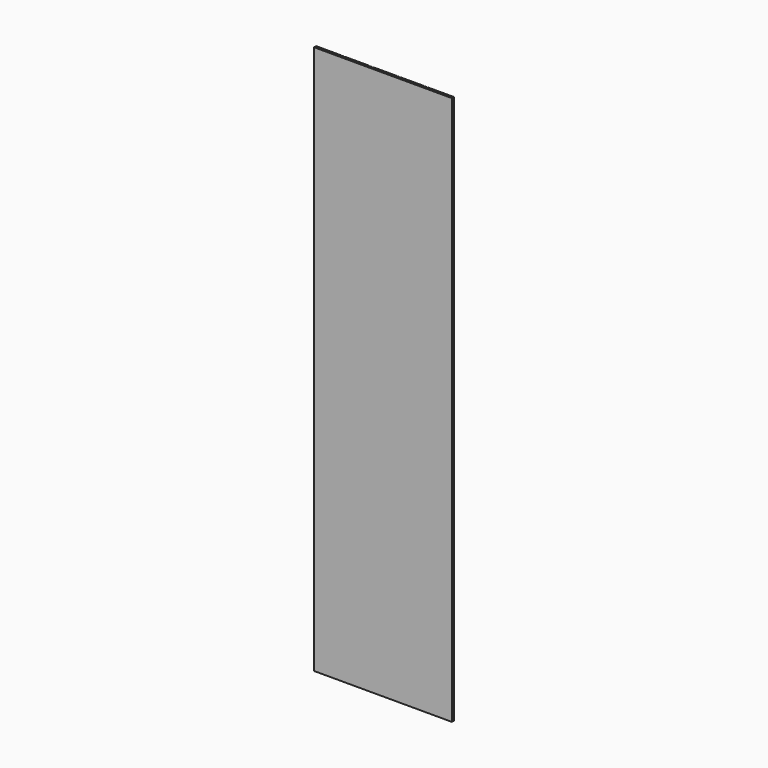
from build123d import *

# Parameters (mm, degrees)
F1_DEPTH = 2390


# Not quite as in the source:
# - a feature names something its author has since deleted; it is built from what else it names


with BuildPart() as f1:
    # F0 (on Top) → F1 (new body)
    with BuildSketch(Plane.XY):
        with BuildLine():
            Line((-309.5, -5.5), (290.5, -5.5))
            ThreePointArc((290.5, -5.5), (285, 0), (290.5, 5.5))
            Line((290.5, 5.5), (180.5, 5.5))
            Line((180.5, 5.5), (176, 0))
            ThreePointArc((176, 0), (170.5, 5.5), (165, 0))
            Line((165, 0), (160.5, 5.5))
            Line((160.5, 5.5), (60.5, 5.5))
            Line((60.5, 5.5), (56, 0))
            ThreePointArc((56, 0), (54.3890872965, 3.8890872965), (50.5, 5.5))
            ThreePointArc((50.5, 5.5), (46.6109127035, 3.8890872965), (45, 0))
            Line((45, 0), (40.5, 5.5))
            Line((40.5, 5.5), (-59.5, 5.5))
            Line((-59.5, 5.5), (-64, 0))
            ThreePointArc((-64, 0), (-65.6109127035, 3.8890872965), (-69.5, 5.5))
            ThreePointArc((-69.5, 5.5), (-73.3890872965, 3.8890872965), (-75, 0))
            Line((-75, 0), (-79.5, 5.5))
            Line((-79.5, 5.5), (-179.5, 5.5))
            Line((-179.5, 5.5), (-184, 0))
            ThreePointArc((-184, 0), (-189.5, 5.5), (-195, 0))
            Line((-195, 0), (-199.5, 5.5))
            Line((-199.5, 5.5), (-309.5, 5.5))
            Line((-309.5, 5.5), (-309.5, -5.5))
        make_face()
        with BuildLine():
            ThreePointArc((290.5, 5.5), (285, 0), (290.5, -5.5))
            Line((290.5, -5.5), (290.5, 5.5))
        make_face()
    extrude(amount=F1_DEPTH)


solid = f1.part
